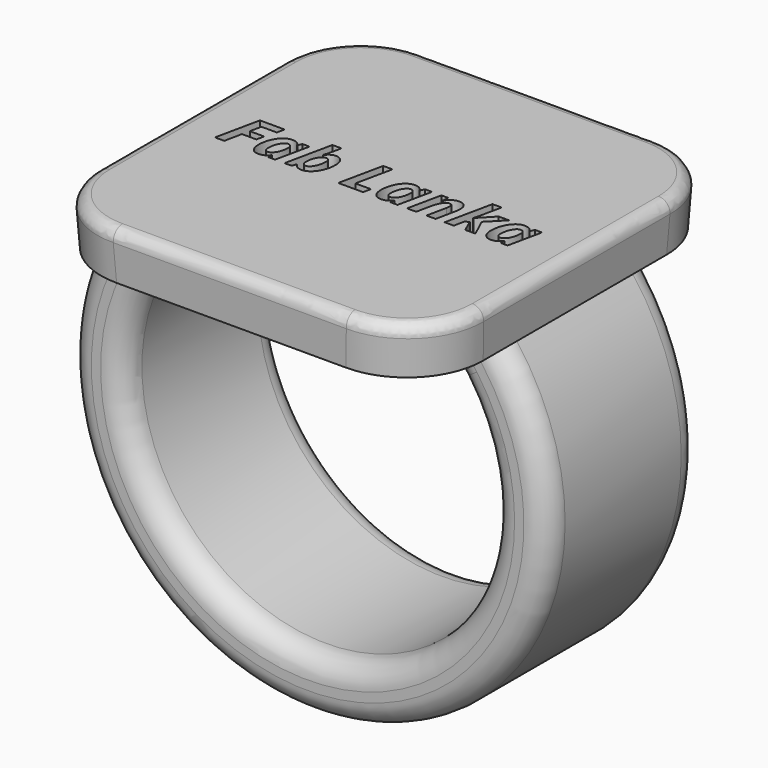
from build123d import *

# Parameters (mm, degrees)
F0_W          = 25.4
F0_H          = 25.4
F1_DEPTH      = 3.175
F1_TAPER      = -3
F3_W          = 5.08
F3_H          = 12.7
F6_DEPTH      = 6.35
F6_DEPTH_BACK = 6.35
F7_R          = 5.08
F8_R          = 1.524
F9_R          = 0.762
F10_TEXT_SIZE = 4.141656051
F11_DEPTH     = 2.032


# Not quite as in the source:
# - Text() gives the source's letters only with a copy of the font that has no kerning and outlines rounded to 1/6400 em; it was checked with that copy


with BuildPart() as f1:
    # F0 (on Top) → F1 (new body)
    with BuildSketch(Plane.XY):
        Rectangle(F0_W, F0_H)
    extrude(amount=F1_DEPTH, taper=F1_TAPER)

    # F4: sweep along a path in F2
    with BuildLine(Plane.XZ) as f4_path:
        ThreePointArc((-10.16, 0), (0, -23.5582897328), (10.16, 0))
    # F3 (on face) → F4 (sweep)
    with BuildSketch(Plane(origin=(0, 0, 0), x_dir=(1, 0, 0), z_dir=(0, 0, -1))):
        with Locations((-10.16, 0)):
            Rectangle(F3_W, F3_H)
    sweep(path=f4_path.line)

    # F5 (on Front) → F6 (join, two sides)
    with BuildSketch(Plane.XZ) as f6_sk:
        with BuildLine():
            ThreePointArc((7.62, 0), (8.9072265211, -1.1822790439), (10.0130578512, -2.535746045))
            Line((10.0130578512, -2.535746045), (10.16, 0))
            Line((10.16, 0), (7.62, 0))
        make_face()
    extrude(amount=F6_DEPTH)
    extrude(f6_sk.sketch, amount=-F6_DEPTH_BACK)

    # F7
    f7_edges = [f1.edges().sort_by_distance(p)[0] for p in [
        (-12.783197, -12.783197, 1.5875),
        (-12.783197, 12.783197, 1.5875),
        (12.783197, 12.783197, 1.5875),
        (12.783197, -12.783197, 1.5875),
    ]]
    fillet(f7_edges, radius=F7_R)

    # F8
    f8_edges = [f1.edges().sort_by_distance(p)[0] for p in [
        (-1.743325, 6.35, -21.711017),
        (8.907227, 6.35, -1.182279),
        (-1.743325, -6.35, -21.711017),
        (8.907227, -6.35, -1.182279),
        (0, 6.35, -25.501344),
        (0, -6.35, -25.501344),
    ]]
    fillet(f8_edges, radius=F8_R)

    # F9
    f9_edges = [f1.edges().sort_by_distance(p)[0] for p in [
        (0, 12.866395, 3.175),
        (11.381378, 11.381378, 3.175),
        (-11.381378, 11.381378, 3.175),
        (12.866395, 0, 3.175),
        (-12.866395, 0, 3.175),
        (11.381378, -11.381378, 3.175),
        (-11.381378, -11.381378, 3.175),
        (0, -12.866395, 3.175),
    ]]
    fillet(f9_edges, radius=F9_R)

    # F10 (on face) → F11 (cut)
    with BuildSketch(Plane.XY.offset(3.175)):
        with Locations((-10.16, -1.4909961783)):
            Text('Fab Lanka', F10_TEXT_SIZE, font='Open Sans', font_style=FontStyle.BOLDITALIC, text_align=(TextAlign.LEFT, TextAlign.BOTTOM))
    extrude(amount=-F11_DEPTH, mode=Mode.SUBTRACT)


solid = f1.part
